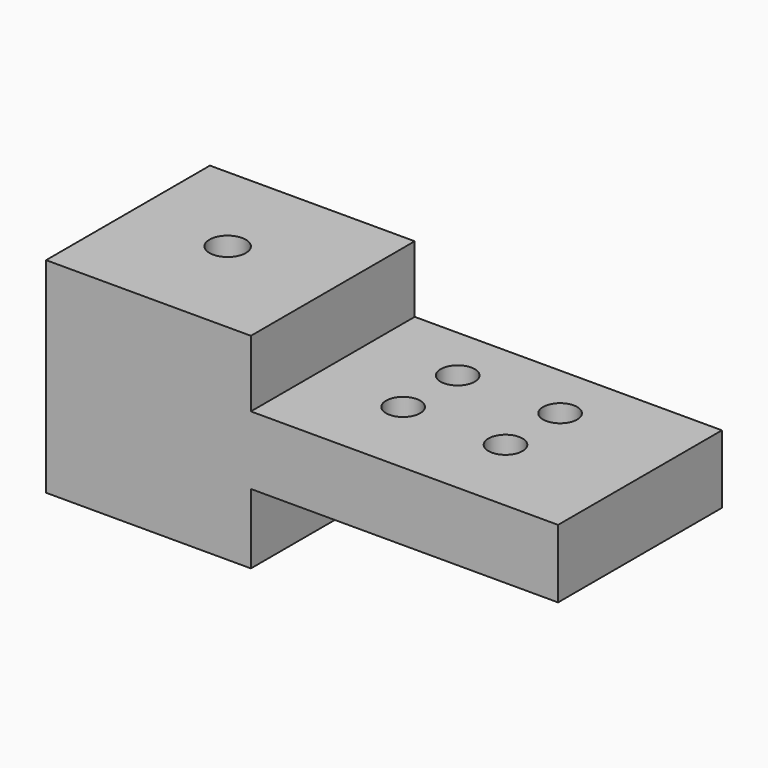
from build123d import *

# Parameters (mm, degrees)
F1_DEPTH = 38.1
F3_D     = 6.7564
F5_D     = 6.35


# Not quite as in the source:
# - the program builds the solid bodies; features that only make, move or delete a surface that nothing else refers to are left out


with BuildPart() as f1:
    # F0 (on Front) → F1 (new body)
    with BuildSketch(Plane.XZ):
        Polygon((0, 38.1), (0, 0), (38.1, 0), (38.1, 13.0175009682), (95.25, 13.0175009682), (95.25, 25.7175009682), (38.1, 25.7175009682), (38.1, 38.1), align=None)
    extrude(amount=F1_DEPTH)

    # F3 (through all)
    with Locations(Plane.XY.offset(38.1)):
        with Locations((17.8784132004, -18.2269066572)):
            Hole(F3_D / 2)

    # F5 (through all)
    with Locations(Plane.XY.offset(25.7175009682)):
        with Locations((54.4917780221, -10.4880234766), (54.4917780221, -23.1880234766), (73.5417780221, -23.1880234766), (73.5417780221, -10.4880234766)):
            Hole(F5_D / 2)


solid = f1.part
